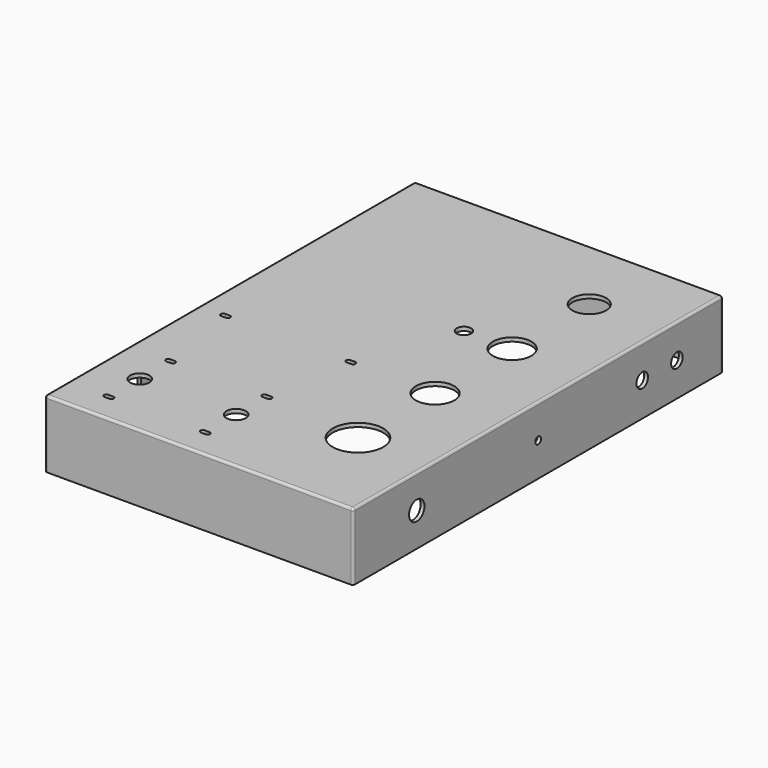
from build123d import *

# Parameters (mm, degrees)
F0_W      = 203.2
F0_H      = 304.8
F1_DEPTH  = 44.45
F2_T      = -2.54
F3_W      = 6.35
F3_H      = 3.175
F4_DEPTH  = 25.4
F5_R      = 1.58749
F7_D      = 33.3375
F7_DEPTH  = 19.05
F7_TIP    = 10.0155954434
F8_D      = 25.4
F8_DEPTH  = 19.05
F8_TIP    = 7.6309298617
F9_D      = 22.225
F9_DEPTH  = 19.05
F9_TIP    = 6.6770636289
F11_D     = 4.7625
F11_DEPTH = 19.05
F11_TIP   = 1.4307993491
F12_D     = 9.525
F12_DEPTH = 19.05
F12_TIP   = 2.8615986981
F13_D     = 12.7
F13_DEPTH = 19.05
F13_TIP   = 3.8154649308
F15_DEPTH = 25.4
F16_D     = 12.7
F16_DEPTH = 19.05
F16_TIP   = 3.8154649308
F17_W     = 6.35
F17_H     = 3.175
F18_DEPTH = 25.4
F19_R     = 1.58749
F20_D     = 9.525
F20_DEPTH = 5.715
F20_TIP   = 2.8615986981
F21_D     = 9.525
F21_DEPTH = 5.715
F21_TIP   = 2.8615986981
F22_R     = 1.5875


# Not quite as in the source:
# - a fillet or chamfer is up to 0.001 mm smaller than in the source, because OpenCascade refuses the exact size


with BuildPart() as f1:
    # F0 (on Top) → F1 (new body)
    with BuildSketch(Plane.XY):
        Rectangle(F0_W, F0_H)
    extrude(amount=F1_DEPTH)

    # F2
    f2_openings = [f1.faces().sort_by_distance(p)[0] for p in [
        (0, 0, 0),
    ]]
    offset(amount=F2_T, openings=f2_openings)

    # F3 (on face) → F4 (cut)
    with BuildSketch(Plane.XY.offset(44.45)):
        with Locations((-74.6125, -133.35)):
            Rectangle(F3_W, F3_H)
        with Locations((-74.6125, -82.55)):
            Rectangle(F3_W, F3_H)
        with Locations((-11.1125, -82.55)):
            Rectangle(F3_W, F3_H)
        with Locations((-11.1125, -133.35)):
            Rectangle(F3_W, F3_H)
    extrude(amount=-F4_DEPTH, mode=Mode.SUBTRACT)

    # F5 (radius 1.5875 in the source; OpenCascade refuses exactly that, so slightly less here)
    f5_edges = [f1.edges().sort_by_distance(p)[0] for p in [
        (-77.7875, -131.7625, 43.18),
        (-14.2875, -131.7625, 43.18),
        (-77.7875, -80.9625, 43.18),
        (-71.4375, -80.9625, 43.18),
        (-7.9375, -80.9625, 43.18),
        (-7.9375, -131.7625, 43.18),
        (-71.4375, -131.7625, 43.18),
        (-14.2875, -134.9375, 43.18),
        (-77.7875, -134.9375, 43.18),
        (-77.7875, -84.1375, 43.18),
        (-14.2875, -84.1375, 43.18),
        (-7.9375, -134.9375, 43.18),
        (-7.9375, -84.1375, 43.18),
        (-71.4375, -84.1375, 43.18),
        (-71.4375, -134.9375, 43.18),
        (-14.2875, -80.9625, 43.18),
    ]]
    fillet(f5_edges, radius=F5_R)

    # F7
    with Locations(Plane.XY.offset(44.45)):
        with Locations((53.975, -88.9)):
            Hole(F7_D / 2, depth=F7_DEPTH)
            with Locations((0, 0, -(F7_DEPTH + F7_TIP / 2))):  # 118° drill point
                Cone(0, F7_D / 2, F7_TIP, mode=Mode.SUBTRACT)

    # F8
    with Locations(Plane.XY.offset(44.45)):
        with Locations((53.975, -25.4), (53.975, 38.1)):
            Hole(F8_D / 2, depth=F8_DEPTH)
            with Locations((0, 0, -(F8_DEPTH + F8_TIP / 2))):  # 118° drill point
                Cone(0, F8_D / 2, F8_TIP, mode=Mode.SUBTRACT)

    # F9
    with Locations(Plane.XY.offset(44.45)):
        with Locations((53.975, 101.6)):
            Hole(F9_D / 2, depth=F9_DEPTH)
            with Locations((0, 0, -(F9_DEPTH + F9_TIP / 2))):  # 118° drill point
                Cone(0, F9_D / 2, F9_TIP, mode=Mode.SUBTRACT)

    # F11
    with Locations(Plane.YZ.offset(101.6)):
        with Locations((0, 22.225)):
            Hole(F11_D / 2, depth=F11_DEPTH)
            with Locations((0, 0, -(F11_DEPTH + F11_TIP / 2))):  # 118° drill point
                Cone(0, F11_D / 2, F11_TIP, mode=Mode.SUBTRACT)

    # F12
    with Locations(Plane.YZ.offset(101.6)):
        with Locations((85.725, 22.225), (114.3, 22.225)):
            Hole(F12_D / 2, depth=F12_DEPTH)
            with Locations((0, 0, -(F12_DEPTH + F12_TIP / 2))):  # 118° drill point
                Cone(0, F12_D / 2, F12_TIP, mode=Mode.SUBTRACT)

    # F13
    with Locations(Plane.YZ.offset(101.6)):
        with Locations((-100.0125, 22.225)):
            Hole(F13_D / 2, depth=F13_DEPTH)
            with Locations((0, 0, -(F13_DEPTH + F13_TIP / 2))):  # 118° drill point
                Cone(0, F13_D / 2, F13_TIP, mode=Mode.SUBTRACT)

    # F14 (on face) → F15 (cut)
    with BuildSketch(Plane(origin=(-101.6, 0, 0), x_dir=(0, -1, 0), z_dir=(-1, 0, 0))):
        Polygon((101.6, 25.5999010921), (96.2436510921, 30.95625), (81.5563489079, 30.95625), (76.2, 25.5999010921), (76.2, 18.8500989079), (81.5563489079, 13.49375), (96.2436510921, 13.49375), (101.6, 18.8500989079), align=None)
        Polygon((81.5563489079, 13.49375), (76.2, 18.8500989079), (76.2, 13.49375), align=None)
        Polygon((101.6, 13.49375), (101.6, 18.8500989079), (96.2436510921, 13.49375), align=None)
    extrude(amount=-F15_DEPTH, mode=Mode.SUBTRACT)

    # F16
    with Locations(Plane.XY.offset(44.45)):
        with Locations((-74.6125, -107.95), (-11.1125, -107.95)):
            Hole(F16_D / 2, depth=F16_DEPTH)
            with Locations((0, 0, -(F16_DEPTH + F16_TIP / 2))):  # 118° drill point
                Cone(0, F16_D / 2, F16_TIP, mode=Mode.SUBTRACT)

    # F17 (on face) → F18 (cut)
    with BuildSketch(Plane.XY.offset(44.45)):
        with Locations((-84.1375, -25.4)):
            Rectangle(F17_W, F17_H)
        with Locations((-1.5875, -25.4)):
            Rectangle(F17_W, F17_H)
    extrude(amount=-F18_DEPTH, mode=Mode.SUBTRACT)

    # F19 (radius 1.5875 in the source; OpenCascade refuses exactly that, so slightly less here)
    f19_edges = [f1.edges().sort_by_distance(p)[0] for p in [
        (-87.3125, -23.8125, 43.18),
        (-4.7625, -23.8125, 43.18),
        (-80.9625, -23.8125, 43.18),
        (1.5875, -23.8125, 43.18),
        (-87.3125, -26.9875, 43.18),
        (-4.7625, -26.9875, 43.18),
        (-80.9625, -26.9875, 43.18),
        (1.5875, -26.9875, 43.18),
    ]]
    fillet(f19_edges, radius=F19_R)

    # F20
    with Locations(Plane(origin=(-101.6, 0, 0), x_dir=(0, -1, 0), z_dir=(-1, 0, 0))):
        with Locations((0, 22.225)):
            Hole(F20_D / 2, depth=F20_DEPTH)
            with Locations((0, 0, -(F20_DEPTH + F20_TIP / 2))):  # 118° drill point
                Cone(0, F20_D / 2, F20_TIP, mode=Mode.SUBTRACT)

    # F21
    with Locations(Plane.XY.offset(44.45)):
        with Locations((22.225, 38.1)):
            Hole(F21_D / 2, depth=F21_DEPTH)
            with Locations((0, 0, -(F21_DEPTH + F21_TIP / 2))):  # 118° drill point
                Cone(0, F21_D / 2, F21_TIP, mode=Mode.SUBTRACT)

    # F22
    f22_edges = [f1.edges().sort_by_distance(p)[0] for p in [
        (0, -152.4, 44.45),
        (101.6, 0, 44.45),
        (101.6, -152.4, 22.225),
        (0, 152.4, 44.45),
        (101.6, 152.4, 22.225),
        (-101.6, 152.4, 22.225),
        (-101.6, 0, 44.45),
        (-101.6, -152.4, 22.225),
    ]]
    fillet(f22_edges, radius=F22_R)


solid = f1.part
